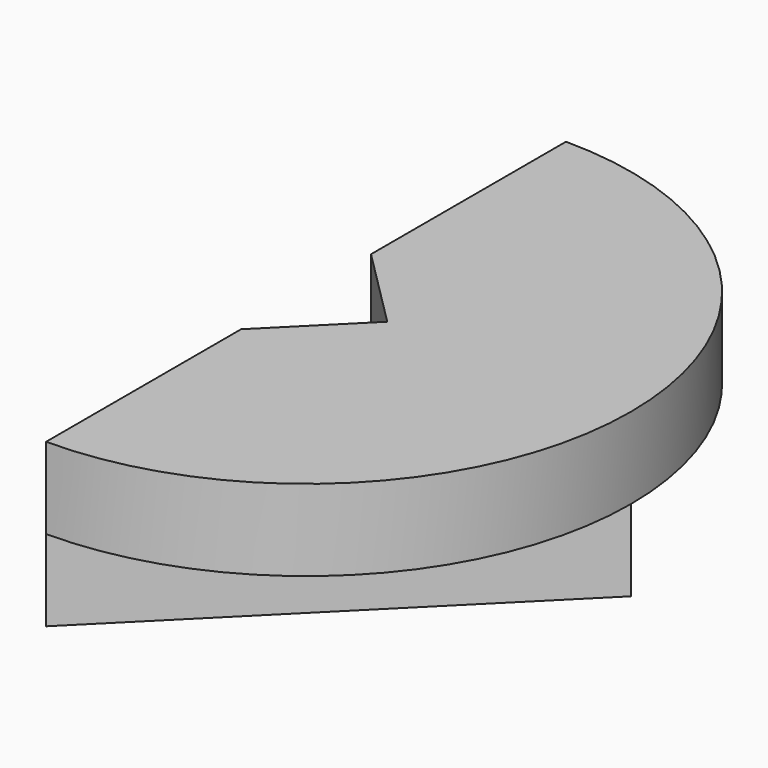
from build123d import *

# Parameters (mm, degrees)
F1_DEPTH = 9.525
F3_DEPTH = 9.525
F5_DEPTH = 25.4
F6_R     = 3.302
F7_DEPTH = 3.175


# Not quite as in the source:
# - a pattern or mirror of a feature is missing from the dataset's text; its kind, count and spacing are read off the source's solid


with BuildPart() as f1:
    # F0 (on Top) → F1 (new body)
    with BuildSketch(Plane.XY):
        Polygon((38.1, 0), (0, 38.1), (0, -38.1), align=None)
    extrude(amount=F1_DEPTH)

    # F2 (on face) → F3 (join)
    with BuildSketch(Plane.XY.offset(9.525)):
        with BuildLine():
            ThreePointArc((0, -38.1), (38.1, 0), (0, 38.1))
            Line((0, 38.1), (0, -38.1))
        make_face()
    extrude(amount=F3_DEPTH)

    # F4 (on face) → F5 (cut)
    with BuildSketch(Plane(origin=(0, 0, 0), x_dir=(1, 0, 0), z_dir=(0, 0, -1))):
        Polygon((9.525, 0), (0, 9.525), (0, -9.525), align=None)
    extrude(amount=-F5_DEPTH, mode=Mode.SUBTRACT)

    # F6 (on face) → F7 (cut)
    with BuildSketch(Plane(origin=(0, 0, 9.525), x_dir=(1, 0, 0), z_dir=(0, 0, -1))):
        with Locations((21.59, 21.59)):
            Circle(F6_R)
    f7 = extrude(amount=-F7_DEPTH, mode=Mode.SUBTRACT)

    # F7_copies: F7 across plane
    add(f7.mirror(Plane.ZX), mode=Mode.SUBTRACT)


solid = f1.part
